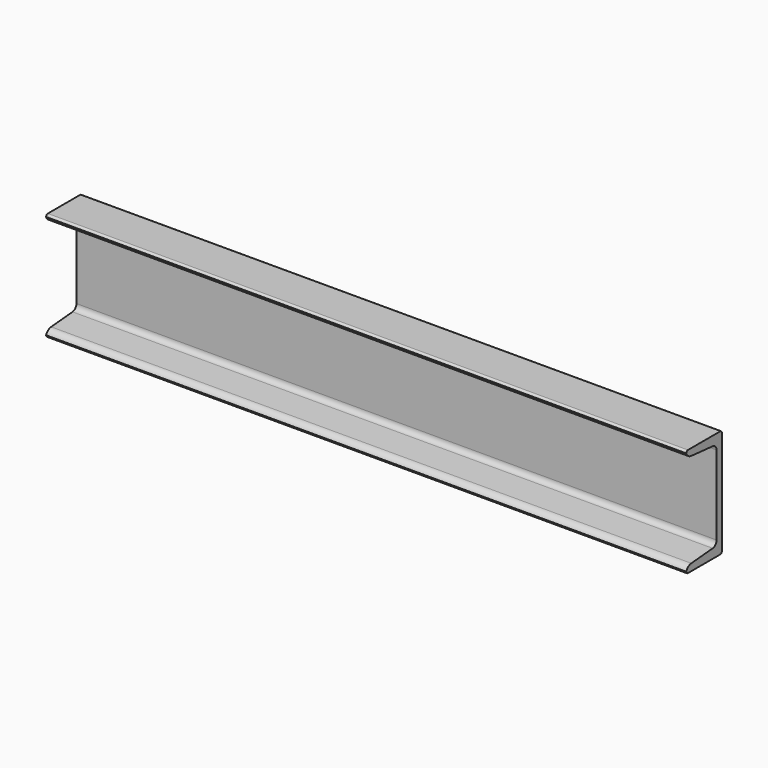
from build123d import *

# Parameters (mm, degrees)
F1_DEPTH    = 300
F2_T1_DEPTH = 629.7738168108


# Not quite as in the source:
# - a fillet or chamfer that OpenCascade refuses, or shapes differently, is made with other operations: its cross-section is extruded or revolved along the edge and cut away or added


with BuildPart() as f1:
    # F0 (on Right) → F1 (new body, symmetric)
    with BuildSketch(Plane.YZ):
        with BuildLine():
            ThreePointArc((-20.915, -48.8), (-20.3292135624, -50.2142135624), (-18.915, -50.8))
            Line((-18.915, -50.8), (18.915, -50.8))
            ThreePointArc((18.915, -50.8), (20.3292135624, -50.2142135624), (20.915, -48.8))
            Line((20.915, -48.8), (20.915, 48.8))
            ThreePointArc((20.915, 48.8), (20.3292135624, 50.2142135624), (18.915, 50.8))
            Line((18.915, 50.8), (-18.915, 50.8))
            ThreePointArc((-18.915, 50.8), (-20.3292135624, 50.2142135624), (-20.915, 48.8))
            Line((-20.915, 48.8), (-20.915, 44.8355484375))
            Line((-20.915, 44.8355484375), (10.0807787137, 42.1237691829))
            ThreePointArc((10.0807787137, 42.1237691829), (13.3313866841, 40.5207467305), (14.645, 37.1427956924))
            Line((14.645, 37.1427956924), (14.645, -37.1427956924))
            ThreePointArc((14.645, -37.1427956924), (13.3313866841, -40.5207467305), (10.0807787137, -42.1237691829))
            Line((10.0807787137, -42.1237691829), (-20.915, -44.8355484375))
            Line((-20.915, -44.8355484375), (-20.915, -48.8))
        make_face()
    extrude(amount=F1_DEPTH, both=True)

    # F2: fillet of radius 7 on 2 edges, made by hand

    # F2_s2 → F2_t1 (cut)
    with BuildSketch(Plane.YZ.offset(-314.8869084054)):
        with BuildLine():
            ThreePointArc((-20.915, -48.8), (-18.5934823683, -45.7054865005), (-14.9828963102, -44.3165566138))
            Line((-14.9828963102, -44.3165566138), (-20.915, -44.8355484375))
            Line((-20.915, -44.8355484375), (-20.915, -48.8))
        make_face()
        with BuildLine():
            ThreePointArc((-14.9828963102, 44.3165566138), (-18.5934823683, 45.7054865005), (-20.915, 48.8))
            Line((-20.915, 48.8), (-20.915, 44.8355484375))
            Line((-20.915, 44.8355484375), (-14.9828963102, 44.3165566138))
        make_face()
    extrude(amount=F2_T1_DEPTH, mode=Mode.SUBTRACT)


solid = f1.part
